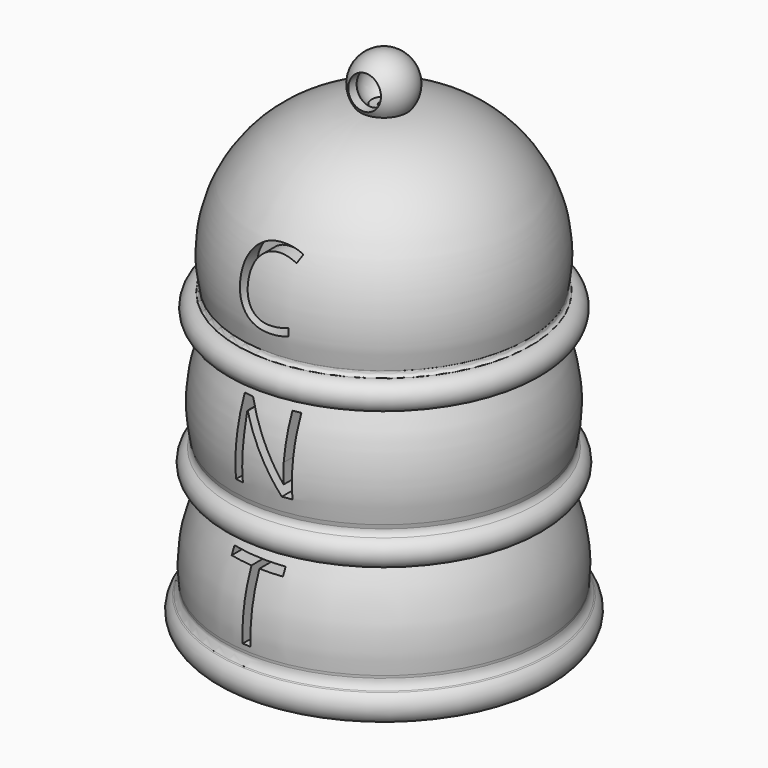
from build123d import *

# Parameters (mm, degrees)
F5_TEXT_SIZE = 6.35
F6_DEPTH     = 3.81
F7_R         = 1.0142492526
F8_DEPTH     = 25.4


# Not quite as in the source:
# - the program builds the solid bodies; features that only make, move or delete a surface that nothing else refers to are left out
# - Text() gives the source's letters only with a copy of the font that has no kerning and outlines rounded to 1/6400 em; it was checked with that copy


with BuildPart() as f3:
    # F2 (on Front) → F3 (revolve)
    with BuildSketch(Plane.XZ):
        with BuildLine():
            ThreePointArc((-31.1364954942, 28.8540312008), (-31.0028583014, 28.7451865193), (-30.9977176919, 28.5729087257))
            ThreePointArc((-30.9977176919, 28.5729087257), (-32.0043172991, 25.9464230361), (-32.1553116571, 23.1377097096))
            ThreePointArc((-32.1553116571, 23.1377097096), (-32.1412764847, 23.0542253432), (-32.1364542145, 22.9697068765))
            ThreePointArc((-32.1364542145, 22.9697068765), (-32.2026226075, 22.6550671506), (-32.3910720383, 22.3945614398))
            ThreePointArc((-32.3910720383, 22.3945614398), (-32.4208422686, 22.3689905159), (-32.4518718733, 22.344963398))
            ThreePointArc((-32.4518718733, 22.344963398), (-32.8187134256, 21.5135278023), (-32.4203744531, 20.6967145205))
            Line((-32.4203744531, 20.6967145205), (-28.4793116152, 20.7101425991))
            ThreePointArc((-28.4793116152, 20.7101425991), (-30.1193645486, 24.9293038108), (-28.4793116152, 29.1484650224))
            ThreePointArc((-28.4793116152, 29.1484650224), (-30.1639912477, 33.5303014144), (-28.4793116152, 37.9121378064))
            ThreePointArc((-28.4793116152, 37.9121378064), (-28.7728033879, 44.9064682258), (-22.3383868426, 47.6641990244))
            Line((-22.3383868426, 47.6641990244), (-22.3383868426, 49.6235868853))
            ThreePointArc((-22.3383868426, 49.6235868853), (-22.5684365507, 49.6389830842), (-22.7988247531, 49.6479934874))
            ThreePointArc((-22.7988247531, 49.6479934874), (-23.3225452384, 51.1563321354), (-22.0373391856, 52.1037570799))
            Line((-22.0373391856, 52.1037570799), (-22.0375297335, 52.6169129437))
            ThreePointArc((-22.0375297335, 52.6169129437), (-23.7019579191, 51.5848261093), (-23.5188517287, 49.6349552055))
            ThreePointArc((-23.5188517287, 49.6349552055), (-29.6514387577, 46.335359439), (-31.1222886718, 39.528557222))
            ThreePointArc((-31.1222886718, 39.528557222), (-31.1203557157, 39.5204900552), (-31.1186624655, 39.512369193))
            ThreePointArc((-31.1186624655, 39.512369193), (-31.1476722153, 39.3253203017), (-31.2890139232, 39.1994180582))
            ThreePointArc((-31.2890139232, 39.1994180582), (-32.0914048996, 38.584662323), (-31.7751951516, 37.6245751977))
            ThreePointArc((-31.7751951516, 37.6245751977), (-31.3839990534, 37.470284403), (-30.9638076524, 37.4535744324))
            ThreePointArc((-30.9638076524, 37.4535744324), (-30.7801684376, 37.3537287936), (-30.8339328108, 37.1517339793))
            ThreePointArc((-30.8339328108, 37.1517339793), (-31.7193946308, 34.2540676166), (-31.5981028357, 31.2265601791))
            ThreePointArc((-31.5981028357, 31.2265601791), (-31.551325496, 31.097172117), (-31.5375928399, 30.9602750599))
            ThreePointArc((-31.5375928399, 30.9602750599), (-31.5885454653, 30.7399729986), (-31.722654581, 30.5579182999))
            ThreePointArc((-31.722654581, 30.5579182999), (-32.2532548226, 29.7510126394), (-31.7382141948, 28.9340876043))
            ThreePointArc((-31.7382141948, 28.9340876043), (-31.5020604365, 28.8701991597), (-31.2583653366, 28.8486810463))
            ThreePointArc((-31.2583653366, 28.8486810463), (-31.1978328677, 28.8605234851), (-31.1364954942, 28.8540312008))
        make_face()
        with BuildLine():
            ThreePointArc((-32.1364542145, 22.9697068765), (-32.1412764847, 23.0542253432), (-32.1553116571, 23.1377097096))
            ThreePointArc((-32.1553116571, 23.1377097096), (-32.1462754992, 23.0536642298), (-32.1364542145, 22.9697068765))
        make_face()
        with BuildLine():
            ThreePointArc((-31.2583653366, 28.8486810463), (-31.197371725, 28.8500192288), (-31.1364954942, 28.8540312008))
            ThreePointArc((-31.1364954942, 28.8540312008), (-31.1978328677, 28.8605234851), (-31.2583653366, 28.8486810463))
        make_face()
        with BuildLine():
            ThreePointArc((-32.4518718733, 22.344963398), (-32.4208422686, 22.3689905159), (-32.3910720383, 22.3945614398))
            ThreePointArc((-32.3910720383, 22.3945614398), (-32.4219229033, 22.3703152136), (-32.4518718733, 22.344963398))
        make_face()
        with BuildLine():
            ThreePointArc((-31.5981028357, 31.2265601791), (-31.568852916, 31.0931892279), (-31.5375928399, 30.9602750599))
            ThreePointArc((-31.5375928399, 30.9602750599), (-31.551325496, 31.097172117), (-31.5981028357, 31.2265601791))
        make_face()
    revolve(axis=Axis((-22.0347086538, 0, 45.019592308), (0.0003713256, 0, -0.9999999311)))

    # F5 (on offset) → F6 (cut)
    with BuildSketch(Plane.XZ.offset(7.62)):
        with Locations((-24.3372886713, 40.7701971867)):
            Text('C', F5_TEXT_SIZE, font='Open Sans', text_align=(TextAlign.LEFT, TextAlign.BOTTOM))
        with Locations((-24.3372886713, 32.1341971867)):
            Text('N', F5_TEXT_SIZE, font='Open Sans', text_align=(TextAlign.LEFT, TextAlign.BOTTOM))
        with Locations((-24.3372886713, 23.4981971867)):
            Text('T', F5_TEXT_SIZE, font='Open Sans', text_align=(TextAlign.LEFT, TextAlign.BOTTOM))
    extrude(amount=F6_DEPTH, mode=Mode.SUBTRACT)

    # F7 (on offset) → F8 (cut)
    with BuildSketch(Plane.XZ.offset(7.62)):
        with Locations((-22.0097694546, 50.9146079421)):
            Circle(F7_R)
    extrude(amount=-F8_DEPTH, mode=Mode.SUBTRACT)


solid = f3.part
